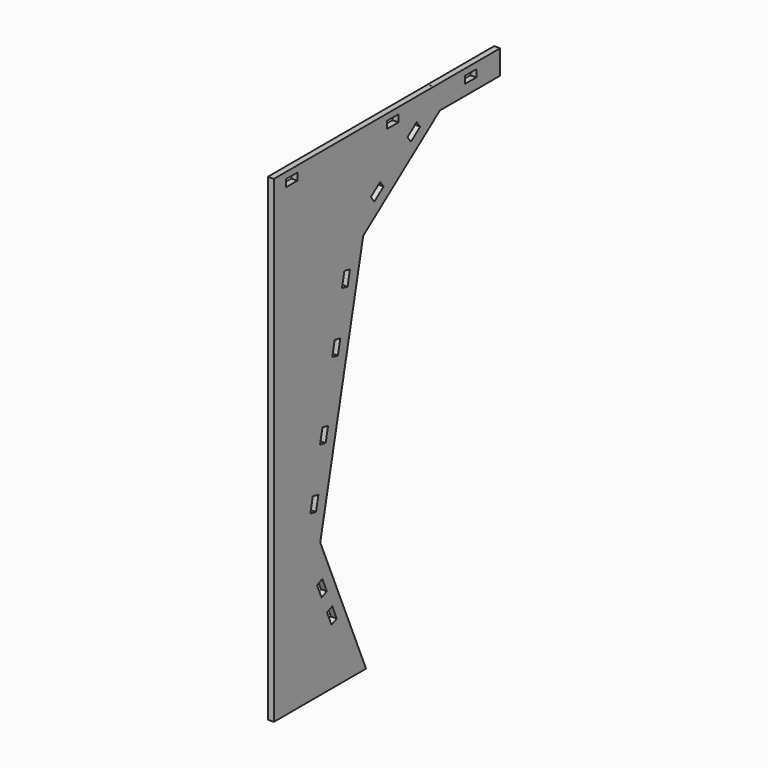
from build123d import *

# Parameters (mm, degrees)
F0_W     = 8.912432854
F0_H     = 0.0079375
F0_W_2   = 2.54
F0_W_3   = 18.0631426697
F1_DEPTH = 2.1082


with BuildPart() as f1:
    # F0 (on Right) → F1 (new body)
    with BuildSketch(Plane.YZ):
        with BuildLine():
            Line((0, 162.0091375), (0, 0))
            Line((0, 0), (12.335197777, 0))
            Line((12.335197777, 0), (18.8042013144, 29.896105485))
            Line((18.8042013144, 29.896105485), (30.5493542935, 2.3257501254))
            Line((30.5493542935, 2.3257501254), (31.5401391658, 0))
            Line((31.5401391658, 0), (31.5707651968, 0))
            Line((31.5707651968, 0), (40.8442968098, 0))
            Line((40.8442968098, 0), (20.5594925834, 47.616175108))
            Line((20.5594925834, 47.616175108), (39.5771112022, 135.5049402038))
            Line((39.5771112022, 135.5049402038), (73.5248959406, 160.7899383022))
            Line((73.5248959406, 160.7899383022), (100.203, 160.7899383022))
            Line((100.203, 160.7899383022), (100.203, 162.0091375))
            Line((100.203, 162.0091375), (82.1398573303, 162.0091375))
            ThreePointArc((82.1398573303, 162.0091375), (80.3438061061, 162.7530862758), (79.5998573303, 164.5491375))
            Line((79.5998573303, 164.5491375), (79.5998573303, 169.3418))
            Line((79.5998573303, 169.3418), (70.6874244764, 169.3418))
            Line((70.6874244764, 169.3418), (70.6874244764, 165.8480664454))
            Line((70.6874244764, 165.8480664454), (70.6874244764, 164.5491375))
            ThreePointArc((70.6874244764, 164.5491375), (70.0510915867, 162.8675752701), (68.4609272063, 162.0285589874))
            ThreePointArc((68.4609272063, 162.0285589874), (68.3044763435, 162.0139975214), (68.1474244764, 162.0091375))
            Line((68.1474244764, 162.0091375), (0, 162.0091375))
        make_face()
        Polygon((21.4843682503, 35.8535070154), (23.4753466245, 31.1799211209), (21.1385536773, 30.1844319338), (19.147575303, 34.8580178283), align=None, mode=Mode.SUBTRACT)
        Polygon((25.8665425285, 25.5668719827), (27.8575209028, 20.8932860882), (25.5207279555, 19.8977969011), (23.5297495813, 24.5713827956), align=None, mode=Mode.SUBTRACT)
        with BuildLine():
            Line((12.3986134924, 50.3752630702), (11.6175919588, 46.7658196656))
            Line((11.6175919588, 46.7658196656), (10.5918, 46.7658196656))
            Line((10.5918, 46.7658196656), (10.5918, 158.7579375))
            Line((10.5918, 158.7579375), (35.8507619547, 158.7579375))
            Line((35.8507619547, 158.7579375), (31.8897708968, 140.4524587956))
            Line((31.8897708968, 140.4524587956), (31.1087493632, 136.8430153909))
            Line((31.1087493632, 136.8430153909), (35.5475592049, 135.882533211))
            ThreePointArc((35.5475592049, 135.882533211), (37.1456481821, 134.7755682604), (37.4929253116, 132.8628062845))
            Line((37.4929253116, 132.8628062845), (29.5595533377, 96.1992113407))
            ThreePointArc((29.5595533377, 96.1992113407), (28.452588387, 94.6011223635), (26.5398264112, 94.2538452339))
            Line((26.5398264112, 94.2538452339), (22.1010165695, 95.2143274138))
            Line((22.1010165695, 95.2143274138), (21.7536814278, 93.6091392306))
            Line((21.7536814278, 93.6091392306), (21.4063462861, 92.0039510473))
            Line((21.4063462861, 92.0039510473), (25.8451561277, 91.0434688674))
            ThreePointArc((25.8451561277, 91.0434688674), (27.4432451049, 89.9365039168), (27.7905222345, 88.0237419409))
            Line((27.7905222345, 88.0237419409), (19.8571502605, 51.3601469971))
            ThreePointArc((19.8571502605, 51.3601469971), (18.7501853099, 49.7620580199), (16.837423334, 49.4147808903))
            Line((16.837423334, 49.4147808903), (12.3986134924, 50.3752630702))
        make_face(mode=Mode.SUBTRACT)
        Polygon((47.0613097153, 149.2568137468), (48.5785484084, 147.2197602993), (44.5044415132, 144.1852829132), (42.9872028202, 146.2223363607), align=None, mode=Mode.SUBTRACT)
        Polygon((44.8088104432, 150.074821282), (46.6876875952, 158.7579375), (56.4668125154, 158.7579375), align=None, mode=Mode.SUBTRACT)
        Polygon((63.2751536106, 161.3332132886), (64.7923923036, 159.296159841), (60.7182854085, 156.2616824549), (59.2010467154, 158.2987359025), align=None, mode=Mode.SUBTRACT)
        with BuildLine():
            Line((0, 164.5491375), (0, 162.0091375))
            Line((0, 162.0091375), (68.1474244764, 162.0091375))
            ThreePointArc((68.1474244764, 162.0091375), (68.3044763435, 162.0139975214), (68.4609272063, 162.0285589874))
            Line((68.4609272063, 162.0285589874), (69.6856973646, 162.9407926238))
            Line((69.6856973646, 162.9407926238), (68.1474244764, 165.0060867035))
            Line((68.1474244764, 165.0060867035), (68.1474244764, 164.5491375))
            Line((68.1474244764, 164.5491375), (55.1748093832, 164.5491375))
            Line((55.1748093832, 164.5491375), (50.0948093832, 164.5491375))
            Line((50.0948093832, 164.5491375), (10.3999171089, 164.5491375))
            Line((10.3999171089, 164.5491375), (5.3199171089, 164.5491375))
            Line((5.3199171089, 164.5491375), (0, 164.5491375))
        make_face()
        Polygon((18.8042013144, 29.896105485), (12.335197777, 0), (13.2072197655, 0), (31.5401391658, 0), (30.5493542935, 2.3257501254), align=None)
        Polygon((0, 169.3418), (0, 164.5491375), (5.3199171089, 164.5491375), (5.3199171089, 167.0891375), (10.3999171089, 167.0891375), (10.3999171089, 164.5491375), (50.0948093832, 164.5491375), (50.0948093832, 167.0891375), (55.1748093832, 167.0891375), (55.1748093832, 164.5491375), (68.1474244764, 164.5491375), (68.1474244764, 165.0060867035), (68.1474244764, 169.3418), align=None)
        with BuildLine():
            Line((69.6856973646, 162.9407926238), (68.4609272063, 162.0285589874))
            ThreePointArc((68.4609272063, 162.0285589874), (70.0510915867, 162.8675752701), (70.6874244764, 164.5491375))
            Line((70.6874244764, 164.5491375), (70.6874244764, 165.8480664454))
            Line((70.6874244764, 165.8480664454), (70.6874244764, 169.3418))
            Line((70.6874244764, 169.3418), (68.1474244764, 169.3418))
            Line((68.1474244764, 169.3418), (68.1474244764, 165.0060867035))
            Line((68.1474244764, 165.0060867035), (69.6856973646, 162.9407926238))
        make_face()
        with Locations((75.1436409033, 169.34576875)):
            Rectangle(F0_W, F0_H)
        with Locations((80.8698573303, 169.34576875)):
            Rectangle(F0_W_2, F0_H)
        with BuildLine():
            Line((82.1398573303, 169.3418), (79.5998573303, 169.3418))
            Line((79.5998573303, 169.3418), (79.5998573303, 164.5491375))
            ThreePointArc((79.5998573303, 164.5491375), (80.3438061061, 162.7530862758), (82.1398573303, 162.0091375))
            Line((82.1398573303, 162.0091375), (100.203, 162.0091375))
            Line((100.203, 162.0091375), (100.203, 164.5491375))
            Line((100.203, 164.5491375), (89.6502663064, 164.5491375))
            Line((89.6502663064, 164.5491375), (84.5702663064, 164.5491375))
            Line((84.5702663064, 164.5491375), (82.1398573303, 164.5491375))
            Line((82.1398573303, 164.5491375), (82.1398573303, 169.3418))
        make_face()
        with Locations((91.1714286652, 169.34576875)):
            Rectangle(F0_W_3, F0_H)
        Polygon((100.203, 169.3418), (82.1398573303, 169.3418), (82.1398573303, 164.5491375), (84.5702663064, 164.5491375), (84.5702663064, 167.0891375), (89.6502663064, 167.0891375), (89.6502663064, 164.5491375), (100.203, 164.5491375), align=None)
        Polygon((10.5918, 46.7658196656), (11.6175919588, 46.7658196656), (12.3986134924, 50.3752630702), (12.9357939022, 52.8578095868), (20.8691658762, 89.5214045307), (21.4063462861, 92.0039510473), (21.7536814278, 93.6091392306), (22.1010165695, 95.2143274138), (22.6381969794, 97.6968739305), (30.5715689534, 134.3604688743), (31.1087493632, 136.8430153909), (31.8897708968, 140.4524587956), (35.8507619547, 158.7579375), (10.5918, 158.7579375), align=None)
        with BuildLine():
            Line((12.9357939022, 52.8578095868), (12.3986134924, 50.3752630702))
            Line((12.3986134924, 50.3752630702), (16.837423334, 49.4147808903))
            ThreePointArc((16.837423334, 49.4147808903), (18.7501853099, 49.7620580199), (19.8571502605, 51.3601469971))
            Line((19.8571502605, 51.3601469971), (27.7905222345, 88.0237419409))
            ThreePointArc((27.7905222345, 88.0237419409), (27.4432451049, 89.9365039168), (25.8451561277, 91.0434688674))
            Line((25.8451561277, 91.0434688674), (21.4063462861, 92.0039510473))
            Line((21.4063462861, 92.0039510473), (20.8691658762, 89.5214045307))
            Line((20.8691658762, 89.5214045307), (25.3079757178, 88.5609223508))
            Line((25.3079757178, 88.5609223508), (24.0175885553, 82.5974767434))
            Line((24.0175885553, 82.5974767434), (22.9432277355, 77.6323837102))
            Line((22.9432277355, 77.6323837102), (19.7419229759, 62.8377489213))
            Line((19.7419229759, 62.8377489213), (18.6675621562, 57.872655888))
            Line((18.6675621562, 57.872655888), (17.3746037439, 51.8973274069))
            Line((17.3746037439, 51.8973274069), (12.9357939022, 52.8578095868))
        make_face()
        Polygon((20.8691658762, 89.5214045307), (12.9357939022, 52.8578095868), (17.3746037439, 51.8973274069), (18.6675621562, 57.872655888), (16.1850156395, 58.4098362979), (17.2593764593, 63.3749293312), (19.7419229759, 62.8377489213), (22.9432277355, 77.6323837102), (20.4606812189, 78.16956412), (21.5350420386, 83.1346571533), (24.0175885553, 82.5974767434), (25.3079757178, 88.5609223508), align=None)
        with BuildLine():
            Line((35.5475592049, 135.882533211), (31.1087493632, 136.8430153909))
            Line((31.1087493632, 136.8430153909), (30.5715689534, 134.3604688743))
            Line((30.5715689534, 134.3604688743), (35.010378795, 133.3999866944))
            Line((35.010378795, 133.3999866944), (33.7174203827, 127.4246582133))
            Line((33.7174203827, 127.4246582133), (32.643059563, 122.45956518))
            Line((32.643059563, 122.45956518), (29.4417548033, 107.6649303911))
            Line((29.4417548033, 107.6649303911), (28.3673939836, 102.6998373579))
            Line((28.3673939836, 102.6998373579), (27.077006821, 96.7363917505))
            Line((27.077006821, 96.7363917505), (22.6381969794, 97.6968739305))
            Line((22.6381969794, 97.6968739305), (22.1010165695, 95.2143274138))
            Line((22.1010165695, 95.2143274138), (26.5398264112, 94.2538452339))
            ThreePointArc((26.5398264112, 94.2538452339), (28.452588387, 94.6011223635), (29.5595533377, 96.1992113407))
            Line((29.5595533377, 96.1992113407), (37.4929253116, 132.8628062845))
            ThreePointArc((37.4929253116, 132.8628062845), (37.1456481821, 134.7755682604), (35.5475592049, 135.882533211))
        make_face()
        Polygon((35.010378795, 133.3999866944), (30.5715689534, 134.3604688743), (22.6381969794, 97.6968739305), (27.077006821, 96.7363917505), (28.3673939836, 102.6998373579), (25.884847467, 103.2370177677), (26.9592082867, 108.202110801), (29.4417548033, 107.6649303911), (32.643059563, 122.45956518), (30.1605130463, 122.9967455899), (31.2348738661, 127.9618386231), (33.7174203827, 127.4246582133), align=None)
        Polygon((56.4668125154, 158.7579375), (46.6876875952, 158.7579375), (44.8088104432, 150.074821282), align=None)
    extrude(amount=F1_DEPTH)


solid = f1.part
